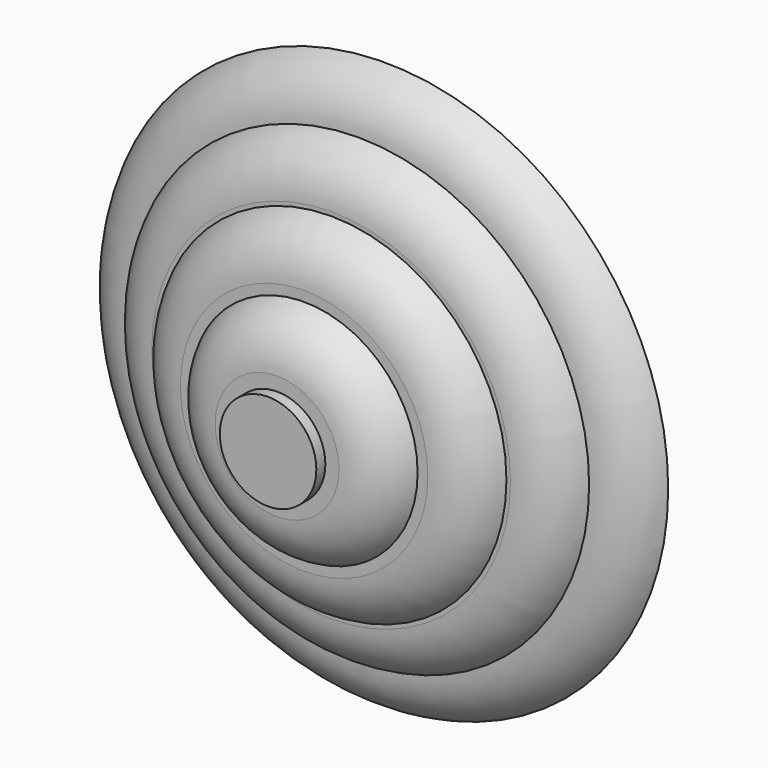
from build123d import *

# Parameters (mm, degrees)
F0_R     = 25.1181711361
F0_R_2   = 20.4995111856
F1_DEPTH = 3
F0_R_3   = 15.560509686
F2_DEPTH = 6
F0_R_4   = 10.0770984701
F3_DEPTH = 9
F0_R_5   = 4.2848341216
F4_DEPTH = 12
F0_R_6   = 1.2539122761
F5_DEPTH = 13
F6_DEPTH = 13


# Not quite as in the source:
# - a fillet or chamfer that OpenCascade refuses, or shapes differently, is made with other operations: its cross-section is extruded or revolved along the edge and cut away or added


with BuildPart() as f1:
    # F0 (on Front) → F1 (new body)
    with BuildSketch(Plane.XZ):
        Circle(F0_R)
        Circle(F0_R_2, mode=Mode.SUBTRACT)
    extrude(amount=F1_DEPTH)

    # F0 (on Front) → F2 (join)
    with BuildSketch(Plane.XZ):
        Circle(F0_R_2)
        Circle(F0_R_3, mode=Mode.SUBTRACT)
    extrude(amount=F2_DEPTH)

    # F0 (on Front) → F3 (join)
    with BuildSketch(Plane.XZ):
        Circle(F0_R_3)
        Circle(F0_R_4, mode=Mode.SUBTRACT)
    extrude(amount=F3_DEPTH)

    # F0 (on Front) → F4 (join)
    with BuildSketch(Plane.XZ):
        Circle(F0_R_4)
        Circle(F0_R_5, mode=Mode.SUBTRACT)
    extrude(amount=F4_DEPTH)

    # F0 (on Front) → F5 (join)
    with BuildSketch(Plane.XZ):
        Circle(F0_R_5)
        Circle(F0_R_6, mode=Mode.SUBTRACT)
    extrude(amount=F5_DEPTH)

    # F0 (on Front) → F6 (join)
    with BuildSketch(Plane.XZ):
        Circle(F0_R_6)
    extrude(amount=F6_DEPTH)

    # F7: fillet of radius 5 on 4 edges, made by hand

    # F7_s1 → F7_t2 (revolve, cut)
    with BuildSketch(Plane.XY):
        with BuildLine():
            ThreePointArc((25.1181711361, 0), (23.2742082286, -2.1833001327), (20.5355954411, -3))
            Line((20.5355954411, -3), (25.1181711361, -3))
            Line((25.1181711361, -3), (25.1181711361, 0))
        make_face()
    revolve(axis=Axis((0, -3, 0), (0, -1, 0)), mode=Mode.SUBTRACT)

    # F7_s3 → F7_t4 (revolve, cut)
    with BuildSketch(Plane.XY):
        with BuildLine():
            ThreePointArc((20.4995111856, -3), (18.6555482782, -5.1833001327), (15.9169354907, -6))
            Line((15.9169354907, -6), (20.4995111856, -6))
            Line((20.4995111856, -6), (20.4995111856, -3))
        make_face()
    revolve(axis=Axis((0, -6, 0), (0, -1, 0)), mode=Mode.SUBTRACT)

    # F7_s5 → F7_t6 (revolve, cut)
    with BuildSketch(Plane.XY):
        with BuildLine():
            ThreePointArc((15.560509686, -6), (13.7165467785, -8.1833001327), (10.977933991, -9))
            Line((10.977933991, -9), (15.560509686, -9))
            Line((15.560509686, -9), (15.560509686, -6))
        make_face()
    revolve(axis=Axis((0, -9, 0), (0, -1, 0)), mode=Mode.SUBTRACT)

    # F7_s7 → F7_t8 (revolve, cut)
    with BuildSketch(Plane.XY):
        with BuildLine():
            ThreePointArc((10.0770984701, -9), (8.2331355627, -11.1833001327), (5.4945227752, -12))
            Line((5.4945227752, -12), (10.0770984701, -12))
            Line((10.0770984701, -12), (10.0770984701, -9))
        make_face()
    revolve(axis=Axis((0, -12, 0), (0, -1, 0)), mode=Mode.SUBTRACT)


solid = f1.part
